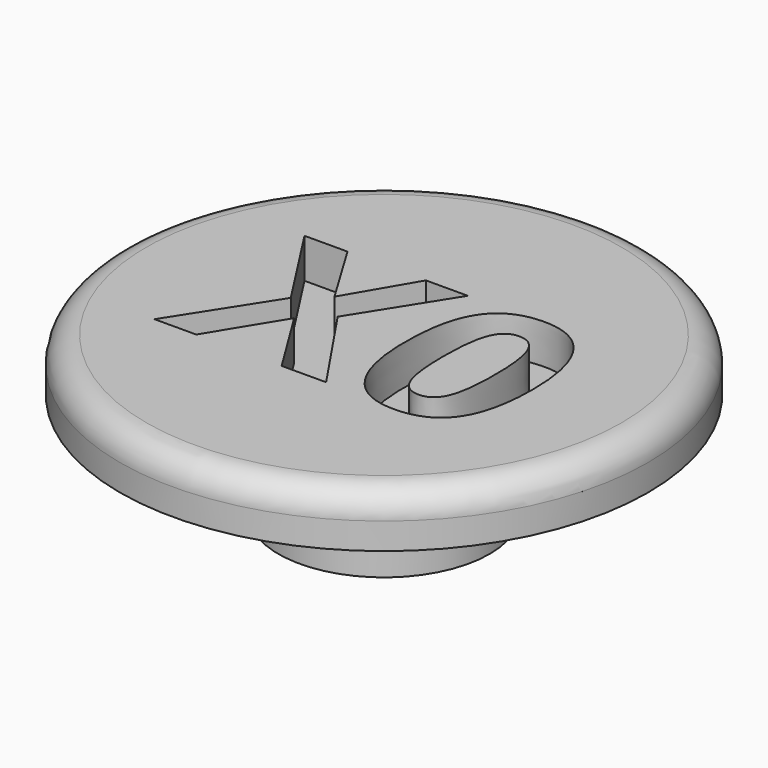
from build123d import *

# Parameters (mm, degrees)
F0_R         = 4
F1_DEPTH     = 6
F0_R_2       = 5
F2_DEPTH     = 2.5
F0_R_3       = 10
F3_DEPTH     = 2
F4_R         = 1
F5_TEXT_SIZE = 9.7222222222
F6_DEPTH     = 1.5


# Not quite as in the source:
# - Text() gives the source's letters only with a copy of the font that has no kerning and outlines rounded to 1/6400 em; it was checked with that copy


with BuildPart() as f1:
    # F0 (on Top) → F1 (new body)
    with BuildSketch(Plane.XY):
        Circle(F0_R)
    extrude(amount=-F1_DEPTH)

    # F0 (on Top) → F2 (join)
    with BuildSketch(Plane.XY):
        Circle(F0_R_2)
        Circle(F0_R, mode=Mode.SUBTRACT)
    extrude(amount=-F2_DEPTH)

    # F0 (on Top) → F3 (join)
    with BuildSketch(Plane.XY):
        Circle(F0_R_3)
        Circle(F0_R_2, mode=Mode.SUBTRACT)
    extrude(amount=-F3_DEPTH)

    # F4
    f4_edges = [f1.edges().sort_by_distance(p)[0] for p in [
        (-10, 0, 0),
    ]]
    fillet(f4_edges, radius=F4_R)

    # F5 (on Top) → F6 (cut)
    with BuildSketch(Plane.XY):
        with Locations(Location((-5.930119755, -3.4506076221), (0, 0, 0.160757428))):
            Text('X', F5_TEXT_SIZE, font='Open Sans', font_style=FontStyle.BOLD, text_align=(TextAlign.LEFT, TextAlign.BOTTOM))
        with Locations((0.4134223001, -3.4306434961)):
            Text('0', F5_TEXT_SIZE, font='Open Sans', font_style=FontStyle.BOLD, text_align=(TextAlign.LEFT, TextAlign.BOTTOM))
    extrude(amount=-F6_DEPTH, mode=Mode.SUBTRACT)


solid = f1.part
